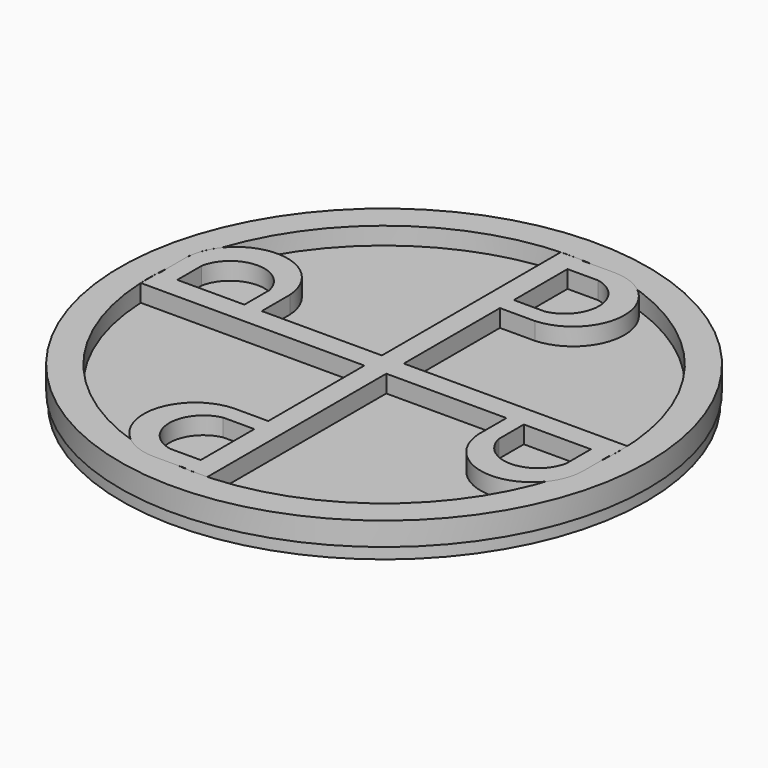
from build123d import *

# Parameters (mm, degrees)
F1_DEPTH = 5.08
F3_COUNT = 4
F4_R     = 57.6415248938
F5_DEPTH = 5.0800000317
F6_R     = 57.3366696562
F7_DEPTH = 2.54
F8_DEPTH = 1.27


with BuildPart() as f1:
    # F0 (on Top) → F1 (new body)
    with BuildSketch(Plane.XY):
        Polygon((-5.2582197823, 28.1538348645), (-10.0426170975, 28.1469915062), (-10.0426170975, -23.0887178332), (-5.2582197823, -23.0887178332), (-5.2582197823, 5.5397343822), (-5.2582197823, 9.3388566747), (-5.2582197823, 23.9849314094), (-5.2582197823, 27.9716439545), align=None)
        with BuildLine():
            Line((1.9807802177, 27.9716439545), (-5.2582197823, 27.9716439545))
            Line((-5.2582197823, 27.9716439545), (-5.2582197823, 23.9849314094))
            Line((-5.2582197823, 23.9849314094), (1.4016701607, 23.9849314094))
            ThreePointArc((1.4016701607, 23.9849314094), (7.4798763217, 16.7329380114), (1.5753391199, 9.3388566747))
            Line((1.5753391199, 9.3388566747), (-5.2582197823, 9.3388566747))
            Line((-5.2582197823, 9.3388566747), (-5.2582197823, 5.5397343822))
            Line((-5.2582197823, 5.5397343822), (2.390121635, 5.5397343822))
            ThreePointArc((2.390121635, 5.5397343822), (12.9688554502, 16.952466624), (1.9807802177, 27.9716439545))
        make_face()
    extrude(amount=F1_DEPTH)


with BuildPart() as f3_1:
    # F3: instance of F1
    add(f1.part.rotate(Axis((-7.6504184399, -23.0887178332, 2.54), (0, 0, -1)), 1 * 360 / F3_COUNT))


with BuildPart() as f3_2:
    # F3: instance of F1
    add(f1.part.rotate(Axis((-7.6504184399, -23.0887178332, 2.54), (0, 0, -1)), 2 * 360 / F3_COUNT))


with BuildPart() as f3_3:
    # F3: instance of F1
    add(f1.part.rotate(Axis((-7.6504184399, -23.0887178332, 2.54), (0, 0, -1)), 3 * 360 / F3_COUNT))


with BuildPart() as f5:
    # F4 (on face) → F5 (new body)
    with BuildSketch(Plane.XY.offset(5.08)):
        with Locations((-7.6504184399, -23.0887178332)):
            Circle(F4_R)
        with BuildLine():
            ThreePointArc((43.6411064539, -23.0887178332), (-6.4539935787, -74.3662869397), (-58.8861277793, -25.4809164908))
            ThreePointArc((-58.8861277793, -25.4809164908), (-58.9418908651, -23.1620825433), (-58.8927614778, -20.8430985631))
            Line((-58.8927614778, -20.8430985631), (-58.8929711375, -20.6965191755))
            Line((-58.8929711375, -20.6965191755), (-58.8861277793, -20.6965191755))
            ThreePointArc((-58.8861277793, -20.6965191755), (-58.8133853302, -19.4594830782), (-58.7107802276, -18.2245652823))
            Line((-58.7107802276, -18.2245652823), (-58.7107802276, -13.4575191755))
            ThreePointArc((-58.7107802276, -13.4575191755), (-58.0376423972, -9.8582625341), (-56.2420833712, -6.6670667248))
            ThreePointArc((-56.2420833712, -6.6670667248), (0.6706372164, 27.5233415864), (43.6411064539, -23.0887178332))
        make_face(mode=Mode.SUBTRACT)
    extrude(amount=-F5_DEPTH)

    # F6 (on face) → F7 (join)
    with BuildSketch(Plane(origin=(0, 0, 0), x_dir=(1, 0, 0), z_dir=(0, 0, -1))):
        with Locations((-7.6504184399, 23.0887178332)):
            Circle(F6_R)
    extrude(amount=F7_DEPTH)


with BuildPart() as f1_1:
    add(f1.part)

    # F8 (add): a face of the model
    f8_faces = [f5.part.faces().sort_by_distance(p)[0] for p in [
        (-7.6873982389, -23.0802766419, 0),
    ]]

    add(f3_1.part)  # F8 merges F3_1

    add(f3_2.part)  # F8 merges F3_2

    add(f3_3.part)  # F8 merges F3_3
    extrude(f8_faces, amount=F8_DEPTH)


solid = Compound([f5.part, f1_1.part])
